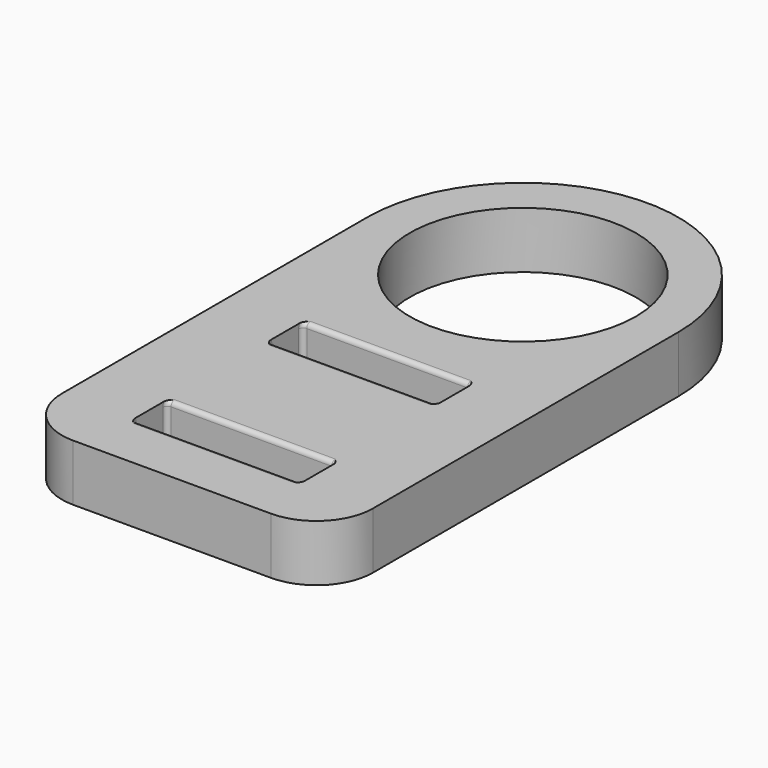
from build123d import *

# Parameters (mm, degrees)
F0_W         = 19.05
F0_H         = 4.7625
F0_R         = 12.7
F1_DEPTH     = 6.35
F2_R         = 0.508
F3_T1_DEPTH  = 5.334
F3_T6_ANGLE  = 233.2969892374
F3_T11_ANGLE = 233.2969892374
F3_T16_ANGLE = 233.2969892374
F3_T21_ANGLE = 233.2969892374
F3_T26_ANGLE = 233.2969892374
F3_T31_ANGLE = 233.2969892374
F3_T36_ANGLE = 233.2969892374
F3_T41_ANGLE = 233.2969892374
F3_T46_ANGLE = 233.2969892374
F3_T51_ANGLE = 233.2969892374
F3_T56_ANGLE = 233.2969892374
F3_T61_ANGLE = 233.2969892374
F3_T66_ANGLE = 233.2969892374
F3_T71_ANGLE = 233.2969892374
F3_T76_ANGLE = 233.2969892374
F3_T81_ANGLE = 233.2969892374


# Not quite as in the source:
# - a fillet or chamfer that OpenCascade refuses, or shapes differently, is made with other operations: its cross-section is extruded or revolved along the edge and cut away or added


with BuildPart() as f1:
    # F0 (on Top) → F1 (new body)
    with BuildSketch(Plane.XY):
        with BuildLine():
            Line((17.4625, -42.8625), (17.4625, 0))
            ThreePointArc((17.4625, 0), (0, 17.4625), (-17.4625, 0))
            Line((-17.4625, 0), (-17.4625, -42.8625))
            ThreePointArc((-17.4625, -42.8625), (-15.6026280605, -47.3526280605), (-11.1125, -49.2125))
            Line((-11.1125, -49.2125), (11.1125, -49.2125))
            ThreePointArc((11.1125, -49.2125), (15.6026280605, -47.3526280605), (17.4625, -42.8625))
        make_face()
        with Locations((0, -40.48125)):
            Rectangle(F0_W, F0_H, mode=Mode.SUBTRACT)
        with Locations((0, -21.43125)):
            Rectangle(F0_W, F0_H, mode=Mode.SUBTRACT)
        Circle(F0_R, mode=Mode.SUBTRACT)
    extrude(amount=F1_DEPTH)

    # F2
    f2_edges = [f1.edges().sort_by_distance(p)[0] for p in [
        (0, -23.8125, 6.35),
        (0, -23.8125, 0),
        (0, -19.05, 6.35),
        (0, -38.1, 6.35),
        (0, -42.8625, 6.35),
        (0, -38.1, 0),
        (0, -19.05, 0),
        (0, -42.8625, 0),
    ]]
    fillet(f2_edges, radius=F2_R)

    # F3: fillet of radius 0.508 on 8 edges, made by hand

    # F3_s2 → F3_t1 (join)
    with BuildSketch(Plane.XY.offset(0.508)):
        with BuildLine():
            ThreePointArc((9.525, -42.3545), (9.3762102448, -42.7137102448), (9.017, -42.8625))
            Line((9.017, -42.8625), (9.525, -42.8625))
            Line((9.525, -42.8625), (9.525, -42.3545))
        make_face()
        with BuildLine():
            ThreePointArc((9.525, -23.3045), (9.3762102448, -23.6637102448), (9.017, -23.8125))
            Line((9.017, -23.8125), (9.525, -23.8125))
            Line((9.525, -23.8125), (9.525, -23.3045))
        make_face()
        with BuildLine():
            ThreePointArc((-9.525, -42.3545), (-9.3762102448, -42.7137102448), (-9.017, -42.8625))
            Line((-9.017, -42.8625), (-9.525, -42.8625))
            Line((-9.525, -42.8625), (-9.525, -42.3545))
        make_face()
        with BuildLine():
            ThreePointArc((9.525, -19.558), (9.3762102448, -19.1987897552), (9.017, -19.05))
            Line((9.017, -19.05), (9.525, -19.05))
            Line((9.525, -19.05), (9.525, -19.558))
        make_face()
        with BuildLine():
            ThreePointArc((-9.525, -19.558), (-9.3762102448, -19.1987897552), (-9.017, -19.05))
            Line((-9.017, -19.05), (-9.525, -19.05))
            Line((-9.525, -19.05), (-9.525, -19.558))
        make_face()
        with BuildLine():
            ThreePointArc((-9.525, -23.3045), (-9.3762102448, -23.6637102448), (-9.017, -23.8125))
            Line((-9.017, -23.8125), (-9.525, -23.8125))
            Line((-9.525, -23.8125), (-9.525, -23.3045))
        make_face()
        with BuildLine():
            ThreePointArc((-9.017, -38.1), (-9.3762102448, -38.2487897552), (-9.525, -38.608))
            Line((-9.525, -38.608), (-9.525, -38.1))
            Line((-9.525, -38.1), (-9.017, -38.1))
        make_face()
        with BuildLine():
            ThreePointArc((9.017, -38.1), (9.3762102448, -38.2487897552), (9.525, -38.608))
            Line((9.525, -38.608), (9.525, -38.1))
            Line((9.525, -38.1), (9.017, -38.1))
        make_face()
    extrude(amount=F3_T1_DEPTH)


with BuildPart() as f3_tool4:
    # F3_s5 → F3_t6 (revolve)
    with BuildSketch(Plane.XY.offset(0.508)):
        with BuildLine():
            ThreePointArc((9.017, -38.1), (9.3762102448, -38.2487897552), (9.525, -38.608))
            Line((9.525, -38.608), (9.525, -38.1))
            Line((9.525, -38.1), (9.017, -38.1))
        make_face()
    revolve(axis=Axis((9.525, -37.592, 0.508), (1, 0, 0)), revolution_arc=F3_T6_ANGLE)

    split(bisect_by=Plane.XY, keep=Keep.TOP)


with BuildPart() as f1_1:
    add(f1.part)

    # F3_t3: union F3_tool4
    add(f3_tool4.part)


with BuildPart() as f3_tool9:
    # F3_s10 → F3_t11 (revolve)
    with BuildSketch(Plane.XY.offset(5.842)):
        with BuildLine():
            ThreePointArc((9.017, -38.1), (9.3762102448, -38.2487897552), (9.525, -38.608))
            Line((9.525, -38.608), (9.525, -38.1))
            Line((9.525, -38.1), (9.017, -38.1))
        make_face()
    revolve(axis=Axis((9.525, -37.592, 5.842), (-1, 0, 0)), revolution_arc=F3_T11_ANGLE)

    split(bisect_by=Plane.XY.offset(6.35), keep=Keep.BOTTOM)


with BuildPart() as f1_2:
    add(f1_1.part)

    # F3_t8: union F3_tool9
    add(f3_tool9.part)


with BuildPart() as f3_tool14:
    # F3_s15 → F3_t16 (revolve)
    with BuildSketch(Plane.XY.offset(0.508)):
        with BuildLine():
            ThreePointArc((-9.525, -38.608), (-9.3762102448, -38.2487897552), (-9.017, -38.1))
            Line((-9.017, -38.1), (-9.525, -38.1))
            Line((-9.525, -38.1), (-9.525, -38.608))
        make_face()
    revolve(axis=Axis((-9.525, -37.592, 0.508), (1, 0, 0)), revolution_arc=F3_T16_ANGLE)

    split(bisect_by=Plane.XY, keep=Keep.TOP)


with BuildPart() as f1_3:
    add(f1_2.part)

    # F3_t13: union F3_tool14
    add(f3_tool14.part)


with BuildPart() as f3_tool19:
    # F3_s20 → F3_t21 (revolve)
    with BuildSketch(Plane.XY.offset(5.842)):
        with BuildLine():
            ThreePointArc((-9.525, -38.608), (-9.3762102448, -38.2487897552), (-9.017, -38.1))
            Line((-9.017, -38.1), (-9.525, -38.1))
            Line((-9.525, -38.1), (-9.525, -38.608))
        make_face()
    revolve(axis=Axis((-9.525, -37.592, 5.842), (-1, 0, 0)), revolution_arc=F3_T21_ANGLE)

    split(bisect_by=Plane.XY.offset(6.35), keep=Keep.BOTTOM)


with BuildPart() as f1_4:
    add(f1_3.part)

    # F3_t18: union F3_tool19
    add(f3_tool19.part)


with BuildPart() as f3_tool24:
    # F3_s25 → F3_t26 (revolve)
    with BuildSketch(Plane.XY.offset(0.508)):
        with BuildLine():
            ThreePointArc((-9.017, -23.8125), (-9.3762102448, -23.6637102448), (-9.525, -23.3045))
            Line((-9.525, -23.3045), (-9.525, -23.8125))
            Line((-9.525, -23.8125), (-9.017, -23.8125))
        make_face()
    revolve(axis=Axis((-9.525, -24.3205, 0.508), (-1, 0, 0)), revolution_arc=F3_T26_ANGLE)

    split(bisect_by=Plane.XY, keep=Keep.TOP)


with BuildPart() as f1_5:
    add(f1_4.part)

    # F3_t23: union F3_tool24
    add(f3_tool24.part)


with BuildPart() as f3_tool29:
    # F3_s30 → F3_t31 (revolve)
    with BuildSketch(Plane.XY.offset(5.842)):
        with BuildLine():
            ThreePointArc((-9.525, -23.3045), (-9.3762102448, -23.6637102448), (-9.017, -23.8125))
            Line((-9.017, -23.8125), (-9.525, -23.8125))
            Line((-9.525, -23.8125), (-9.525, -23.3045))
        make_face()
    revolve(axis=Axis((-9.525, -24.3205, 5.842), (1, 0, 0)), revolution_arc=F3_T31_ANGLE)

    split(bisect_by=Plane.XY.offset(6.35), keep=Keep.BOTTOM)


with BuildPart() as f1_6:
    add(f1_5.part)

    # F3_t28: union F3_tool29
    add(f3_tool29.part)


with BuildPart() as f3_tool34:
    # F3_s35 → F3_t36 (revolve)
    with BuildSketch(Plane.XY.offset(0.508)):
        with BuildLine():
            ThreePointArc((-9.525, -19.558), (-9.3762102448, -19.1987897552), (-9.017, -19.05))
            Line((-9.017, -19.05), (-9.525, -19.05))
            Line((-9.525, -19.05), (-9.525, -19.558))
        make_face()
    revolve(axis=Axis((-9.525, -18.542, 0.508), (1, 0, 0)), revolution_arc=F3_T36_ANGLE)

    split(bisect_by=Plane.XY, keep=Keep.TOP)


with BuildPart() as f1_7:
    add(f1_6.part)

    # F3_t33: union F3_tool34
    add(f3_tool34.part)


with BuildPart() as f3_tool39:
    # F3_s40 → F3_t41 (revolve)
    with BuildSketch(Plane.XY.offset(5.842)):
        with BuildLine():
            ThreePointArc((-9.525, -19.558), (-9.3762102448, -19.1987897552), (-9.017, -19.05))
            Line((-9.017, -19.05), (-9.525, -19.05))
            Line((-9.525, -19.05), (-9.525, -19.558))
        make_face()
    revolve(axis=Axis((-9.525, -18.542, 5.842), (-1, 0, 0)), revolution_arc=F3_T41_ANGLE)

    split(bisect_by=Plane.XY.offset(6.35), keep=Keep.BOTTOM)


with BuildPart() as f1_8:
    add(f1_7.part)

    # F3_t38: union F3_tool39
    add(f3_tool39.part)


with BuildPart() as f3_tool44:
    # F3_s45 → F3_t46 (revolve)
    with BuildSketch(Plane.XY.offset(0.508)):
        with BuildLine():
            ThreePointArc((9.525, -19.558), (9.3762102448, -19.1987897552), (9.017, -19.05))
            Line((9.017, -19.05), (9.525, -19.05))
            Line((9.525, -19.05), (9.525, -19.558))
        make_face()
    revolve(axis=Axis((9.525, -18.542, 0.508), (1, 0, 0)), revolution_arc=F3_T46_ANGLE)

    split(bisect_by=Plane.XY, keep=Keep.TOP)


with BuildPart() as f1_9:
    add(f1_8.part)

    # F3_t43: union F3_tool44
    add(f3_tool44.part)


with BuildPart() as f3_tool49:
    # F3_s50 → F3_t51 (revolve)
    with BuildSketch(Plane.XY.offset(5.842)):
        with BuildLine():
            ThreePointArc((9.525, -19.558), (9.3762102448, -19.1987897552), (9.017, -19.05))
            Line((9.017, -19.05), (9.525, -19.05))
            Line((9.525, -19.05), (9.525, -19.558))
        make_face()
    revolve(axis=Axis((9.525, -18.542, 5.842), (-1, 0, 0)), revolution_arc=F3_T51_ANGLE)

    split(bisect_by=Plane.XY.offset(6.35), keep=Keep.BOTTOM)


with BuildPart() as f1_10:
    add(f1_9.part)

    # F3_t48: union F3_tool49
    add(f3_tool49.part)


with BuildPart() as f3_tool54:
    # F3_s55 → F3_t56 (revolve)
    with BuildSketch(Plane.XY.offset(0.508)):
        with BuildLine():
            ThreePointArc((-9.525, -42.3545), (-9.3762102448, -42.7137102448), (-9.017, -42.8625))
            Line((-9.017, -42.8625), (-9.525, -42.8625))
            Line((-9.525, -42.8625), (-9.525, -42.3545))
        make_face()
    revolve(axis=Axis((-9.525, -43.3705, 0.508), (-1, 0, 0)), revolution_arc=F3_T56_ANGLE)

    split(bisect_by=Plane.XY, keep=Keep.TOP)


with BuildPart() as f1_11:
    add(f1_10.part)

    # F3_t53: union F3_tool54
    add(f3_tool54.part)


with BuildPart() as f3_tool59:
    # F3_s60 → F3_t61 (revolve)
    with BuildSketch(Plane.XY.offset(5.842)):
        with BuildLine():
            ThreePointArc((-9.525, -42.3545), (-9.3762102448, -42.7137102448), (-9.017, -42.8625))
            Line((-9.017, -42.8625), (-9.525, -42.8625))
            Line((-9.525, -42.8625), (-9.525, -42.3545))
        make_face()
    revolve(axis=Axis((-9.525, -43.3705, 5.842), (1, 0, 0)), revolution_arc=F3_T61_ANGLE)

    split(bisect_by=Plane.XY.offset(6.35), keep=Keep.BOTTOM)


with BuildPart() as f1_12:
    add(f1_11.part)

    # F3_t58: union F3_tool59
    add(f3_tool59.part)


with BuildPart() as f3_tool64:
    # F3_s65 → F3_t66 (revolve)
    with BuildSketch(Plane.XY.offset(0.508)):
        with BuildLine():
            ThreePointArc((9.525, -23.3045), (9.3762102448, -23.6637102448), (9.017, -23.8125))
            Line((9.017, -23.8125), (9.525, -23.8125))
            Line((9.525, -23.8125), (9.525, -23.3045))
        make_face()
    revolve(axis=Axis((9.525, -24.3205, 0.508), (-1, 0, 0)), revolution_arc=F3_T66_ANGLE)

    split(bisect_by=Plane.XY, keep=Keep.TOP)


with BuildPart() as f1_13:
    add(f1_12.part)

    # F3_t63: union F3_tool64
    add(f3_tool64.part)


with BuildPart() as f3_tool69:
    # F3_s70 → F3_t71 (revolve)
    with BuildSketch(Plane.XY.offset(5.842)):
        with BuildLine():
            ThreePointArc((9.525, -23.3045), (9.3762102448, -23.6637102448), (9.017, -23.8125))
            Line((9.017, -23.8125), (9.525, -23.8125))
            Line((9.525, -23.8125), (9.525, -23.3045))
        make_face()
    revolve(axis=Axis((9.525, -24.3205, 5.842), (1, 0, 0)), revolution_arc=F3_T71_ANGLE)

    split(bisect_by=Plane.XY.offset(6.35), keep=Keep.BOTTOM)


with BuildPart() as f1_14:
    add(f1_13.part)

    # F3_t68: union F3_tool69
    add(f3_tool69.part)


with BuildPart() as f3_tool74:
    # F3_s75 → F3_t76 (revolve)
    with BuildSketch(Plane.XY.offset(0.508)):
        with BuildLine():
            ThreePointArc((9.525, -42.3545), (9.3762102448, -42.7137102448), (9.017, -42.8625))
            Line((9.017, -42.8625), (9.525, -42.8625))
            Line((9.525, -42.8625), (9.525, -42.3545))
        make_face()
    revolve(axis=Axis((9.525, -43.3705, 0.508), (-1, 0, 0)), revolution_arc=F3_T76_ANGLE)

    split(bisect_by=Plane.XY, keep=Keep.TOP)


with BuildPart() as f1_15:
    add(f1_14.part)

    # F3_t73: union F3_tool74
    add(f3_tool74.part)


with BuildPart() as f3_tool79:
    # F3_s80 → F3_t81 (revolve)
    with BuildSketch(Plane.XY.offset(5.842)):
        with BuildLine():
            ThreePointArc((9.525, -42.3545), (9.3762102448, -42.7137102448), (9.017, -42.8625))
            Line((9.017, -42.8625), (9.525, -42.8625))
            Line((9.525, -42.8625), (9.525, -42.3545))
        make_face()
    revolve(axis=Axis((9.525, -43.3705, 5.842), (1, 0, 0)), revolution_arc=F3_T81_ANGLE)

    split(bisect_by=Plane.XY.offset(6.35), keep=Keep.BOTTOM)


with BuildPart() as f1_16:
    add(f1_15.part)

    # F3_t78: union F3_tool79
    add(f3_tool79.part)


solid = f1_16.part
